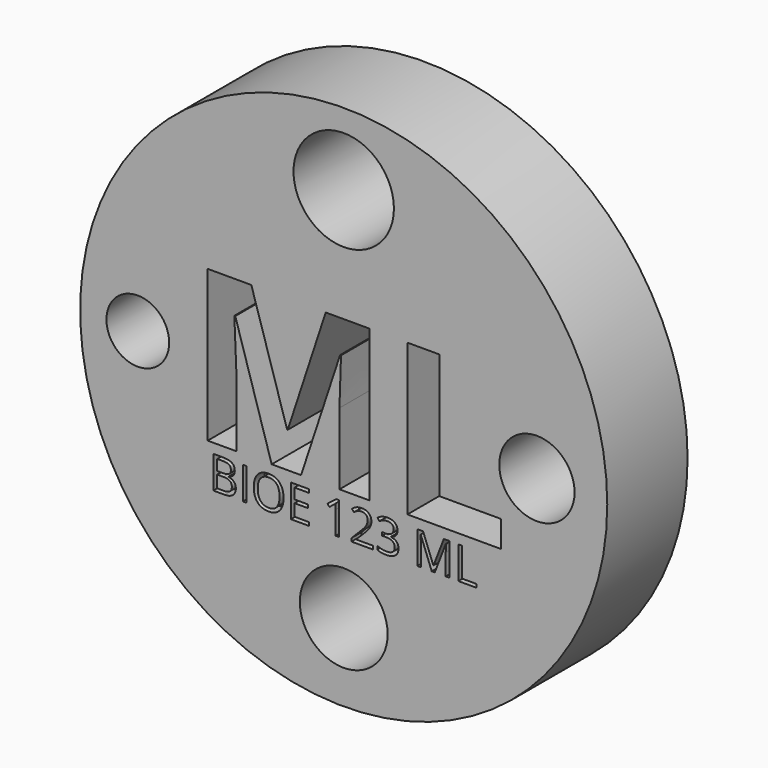
from build123d import *

# Parameters (mm, degrees)
F0_R         = 21
F3_DEPTH     = 8
F1_TEXT_SIZE = 16.8797456556
F4_DEPTH     = 8
F2_R         = 4
F2_R_2       = 3.5
F2_R_3       = 3
F2_R_4       = 2.5
F5_DEPTH     = 8
F6_TEXT_SIZE = 3.6148005165
F7_DEPTH     = 1


# Not quite as in the source:
# - Text() gives the source's letters only with a copy of the font that has no kerning and outlines rounded to 1/6400 em; it was checked with that copy


with BuildPart() as f3:
    # F0 (on Front) → F3 (new body)
    with BuildSketch(Plane.XZ):
        Circle(F0_R)
    extrude(amount=F3_DEPTH)

    # F1 (on Front) → F4 (cut)
    with BuildSketch(Plane.XZ):
        with Locations((-12.3559758067, -5.8741508983)):
            Text('ML', F1_TEXT_SIZE, font='Open Sans', font_style=FontStyle.BOLD, text_align=(TextAlign.LEFT, TextAlign.BOTTOM))
    extrude(amount=F4_DEPTH, mode=Mode.SUBTRACT)

    # F2 (on Front) → F5 (cut)
    with BuildSketch(Plane.XZ):
        with Locations((0, 15.2303539217)):
            Circle(F2_R)
        with Locations((0, -14.7866588086)):
            Circle(F2_R_2)
        with Locations((15.3943300247, 0)):
            Circle(F2_R_3)
        with Locations((-16.4071135223, 0)):
            Circle(F2_R_4)
    extrude(amount=F5_DEPTH, mode=Mode.SUBTRACT)

    # F6 (on face) → F7 (cut)
    with BuildSketch(Plane.XZ.offset(8)):
        with Locations((-10.7370400801, -9.2296414077)):
            Text('BIOE 123 ML', F6_TEXT_SIZE, font='Open Sans', text_align=(TextAlign.LEFT, TextAlign.BOTTOM))
    extrude(amount=-F7_DEPTH, mode=Mode.SUBTRACT)


solid = f3.part
